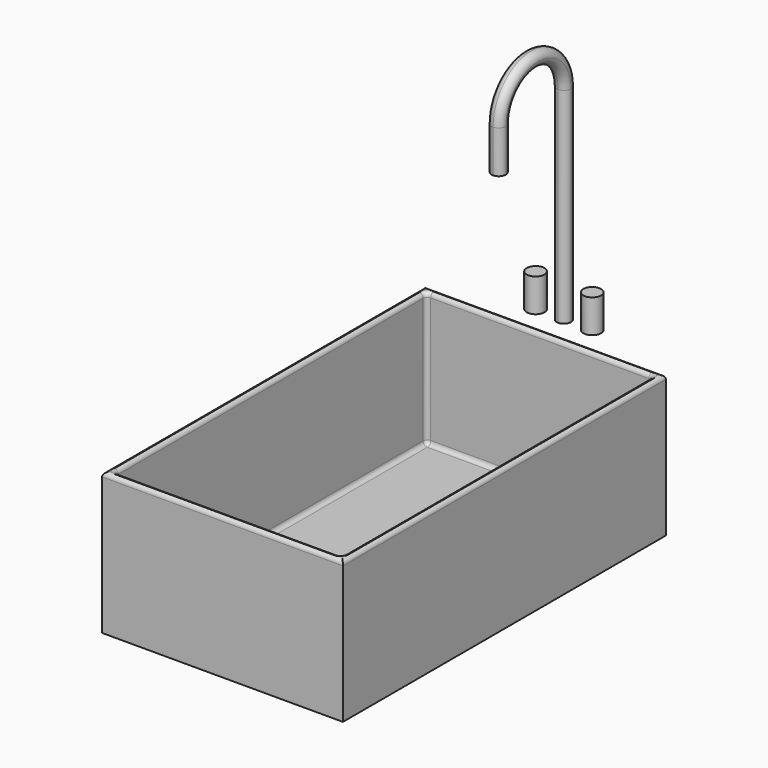
from build123d import *

# Parameters (mm, degrees)
F0_W         = 340
F0_H         = 570
F0_W_2       = 320
F0_H_2       = 550
F1_DEPTH     = 200
F2_W         = 340
F2_H         = 10.8207641169
F3_DEPTH     = 570
F4_T1_DEPTH  = 538
F4_T3_DEPTH  = 308
F4_T5_DEPTH  = 183.1792358831
F4_S9_W      = 6
F4_S9_H      = 6
F4_T10_DEPTH = 6
F4_S15_W     = 6
F4_S15_H     = 6
F4_T16_DEPTH = 6
F4_S21_W     = 6
F4_S21_H     = 6
F4_T22_DEPTH = 6
F4_S27_W     = 6
F4_S27_H     = 6
F4_T28_DEPTH = 6
F4_T31_DEPTH = 600
F4_T33_DEPTH = 370
F4_T35_DEPTH = 538
F4_T37_DEPTH = 308
F4_T40_ANGLE = 90
F4_T42_ANGLE = 90
F4_T44_ANGLE = 90
F4_T46_ANGLE = 90
F5_R         = 14.5871340725
F6_DEPTH     = 3
F12_R        = 12.5
F13_DEPTH    = 47


# Not quite as in the source:
# - a fillet or chamfer that OpenCascade refuses, or shapes differently, is made with other operations: its cross-section is extruded or revolved along the edge and cut away or added


with BuildPart() as f1:
    # F0 (on Top) → F1 (new body)
    with BuildSketch(Plane.XY):
        with Locations((152.4177306145, 254.675924629)):
            Rectangle(F0_W, F0_H)
        with Locations((152.4177306145, 254.675924629)):
            Rectangle(F0_W_2, F0_H_2, mode=Mode.SUBTRACT)
    extrude(amount=F1_DEPTH)

    # F2 (on face) → F3 (join, through all)
    with BuildSketch(Plane.XZ.offset(30.324075371)):
        with Locations((152.4177306145, 5.4103820585)):
            Rectangle(F2_W, F2_H)
    extrude(amount=-F3_DEPTH)

    # F4: fillet of radius 6 on 16 edges, made by hand

    # F4_s2 → F4_t1 (join)
    with BuildSketch(Plane.XZ.offset(-523.675924629)):
        with BuildLine():
            ThreePointArc((-1.5822693855, 10.8207641169), (-5.8249100726, 12.5781234298), (-7.5822693855, 16.8207641169))
            Line((-7.5822693855, 16.8207641169), (-7.5822693855, 10.8207641169))
            Line((-7.5822693855, 10.8207641169), (-1.5822693855, 10.8207641169))
        make_face()
        with BuildLine():
            ThreePointArc((306.4177306145, 10.8207641169), (310.6603713017, 12.5781234298), (312.4177306145, 16.8207641169))
            Line((312.4177306145, 16.8207641169), (312.4177306145, 10.8207641169))
            Line((312.4177306145, 10.8207641169), (306.4177306145, 10.8207641169))
        make_face()
    extrude(amount=F4_T1_DEPTH)

    # F4_s4 → F4_t3 (join)
    with BuildSketch(Plane.YZ.offset(-1.5822693855)):
        with BuildLine():
            ThreePointArc((523.675924629, 10.8207641169), (527.9185653161, 12.5781234298), (529.675924629, 16.8207641169))
            Line((529.675924629, 16.8207641169), (529.675924629, 10.8207641169))
            Line((529.675924629, 10.8207641169), (523.675924629, 10.8207641169))
        make_face()
        with BuildLine():
            ThreePointArc((-20.324075371, 16.8207641169), (-18.5667160581, 12.5781234298), (-14.324075371, 10.8207641169))
            Line((-14.324075371, 10.8207641169), (-20.324075371, 10.8207641169))
            Line((-20.324075371, 10.8207641169), (-20.324075371, 16.8207641169))
        make_face()
    extrude(amount=F4_T3_DEPTH)

    # F4_s6 → F4_t5 (join)
    with BuildSketch(Plane.XY.offset(16.8207641169)):
        with BuildLine():
            ThreePointArc((312.4177306145, 523.675924629), (310.6603713017, 527.9185653161), (306.4177306145, 529.675924629))
            Line((306.4177306145, 529.675924629), (312.4177306145, 529.675924629))
            Line((312.4177306145, 529.675924629), (312.4177306145, 523.675924629))
        make_face()
        with BuildLine():
            ThreePointArc((-1.5822693855, 529.675924629), (-5.8249100726, 527.9185653161), (-7.5822693855, 523.675924629))
            Line((-7.5822693855, 523.675924629), (-7.5822693855, 529.675924629))
            Line((-7.5822693855, 529.675924629), (-1.5822693855, 529.675924629))
        make_face()
        with BuildLine():
            ThreePointArc((-1.5822693855, -20.324075371), (-5.8249100726, -18.5667160581), (-7.5822693855, -14.324075371))
            Line((-7.5822693855, -14.324075371), (-7.5822693855, -20.324075371))
            Line((-7.5822693855, -20.324075371), (-1.5822693855, -20.324075371))
        make_face()
        with BuildLine():
            ThreePointArc((306.4177306145, -20.324075371), (310.6603713017, -18.5667160581), (312.4177306145, -14.324075371))
            Line((312.4177306145, -14.324075371), (312.4177306145, -20.324075371))
            Line((312.4177306145, -20.324075371), (306.4177306145, -20.324075371))
        make_face()
    extrude(amount=F4_T5_DEPTH)


with BuildPart() as f4_tool8:
    # F4_s9 → F4_t10 (new body)
    with BuildSketch(Plane.YZ.offset(-1.5822693855)):
        with Locations((-17.324075371, 13.8207641169)):
            Rectangle(F4_S9_W, F4_S9_H)
    extrude(amount=-F4_T10_DEPTH)

    # F4_s11 → F4_t12 (revolve, cut)
    with BuildSketch(Plane(origin=(-1.5822693855, -14.324075371, 16.8207641169), x_dir=(0, 0.7071067812, 0.7071067812), z_dir=(0, -0.7071067812, 0.7071067812))):
        with BuildLine():
            ThreePointArc((0, -6), (6, 0), (0, 6))
            Line((0, 6), (0, -6))
        make_face()
    revolve(axis=Axis((-1.5822693855, -14.324075371, 16.8207641169), (-1, 0, 0)), mode=Mode.SUBTRACT)


with BuildPart() as f1_1:
    add(f1.part)

    # F4_t7: union F4_tool8
    add(f4_tool8.part)


with BuildPart() as f4_tool14:
    # F4_s15 → F4_t16 (new body)
    with BuildSketch(Plane.YZ.offset(-1.5822693855)):
        with Locations((526.675924629, 13.8207641169)):
            Rectangle(F4_S15_W, F4_S15_H)
    extrude(amount=-F4_T16_DEPTH)

    # F4_s17 → F4_t18 (revolve, cut)
    with BuildSketch(Plane(origin=(-1.5822693855, 523.675924629, 16.8207641169), x_dir=(0, -0.7071067812, 0.7071067812), z_dir=(0, -0.7071067812, -0.7071067812))):
        with BuildLine():
            ThreePointArc((0, -6), (6, 0), (0, 6))
            Line((0, 6), (0, -6))
        make_face()
    revolve(axis=Axis((-1.5822693855, 523.675924629, 16.8207641169), (-1, 0, 0)), mode=Mode.SUBTRACT)


with BuildPart() as f1_2:
    add(f1_1.part)

    # F4_t13: union F4_tool14
    add(f4_tool14.part)


with BuildPart() as f4_tool20:
    # F4_s21 → F4_t22 (new body)
    with BuildSketch(Plane.XY.offset(16.8207641169)):
        with Locations((309.4177306145, 526.675924629)):
            Rectangle(F4_S21_W, F4_S21_H)
    extrude(amount=-F4_T22_DEPTH)

    # F4_s23 → F4_t24 (revolve, cut)
    with BuildSketch(Plane(origin=(306.4177306145, 523.675924629, 16.8207641169), x_dir=(-0.7071067812, -0.7071067812, 0), z_dir=(0.7071067812, -0.7071067812, 0))):
        with BuildLine():
            ThreePointArc((0, -6), (6, 0), (0, 6))
            Line((0, 6), (0, -6))
        make_face()
    revolve(axis=Axis((306.4177306145, 523.675924629, 16.8207641169), (0, 0, -1)), mode=Mode.SUBTRACT)


with BuildPart() as f1_3:
    add(f1_2.part)

    # F4_t19: union F4_tool20
    add(f4_tool20.part)


with BuildPart() as f4_tool26:
    # F4_s27 → F4_t28 (new body)
    with BuildSketch(Plane.XZ.offset(14.324075371)):
        with Locations((309.4177306145, 13.8207641169)):
            Rectangle(F4_S27_W, F4_S27_H)
    extrude(amount=F4_T28_DEPTH)

    # F4_s29 → F4_t30 (revolve, cut)
    with BuildSketch(Plane(origin=(306.4177306145, -14.324075371, 16.8207641169), x_dir=(-0.7071067812, 0, 0.7071067812), z_dir=(0.7071067812, 0, 0.7071067812))):
        with BuildLine():
            ThreePointArc((0, -6), (6, 0), (0, 6))
            Line((0, 6), (0, -6))
        make_face()
    revolve(axis=Axis((306.4177306145, -14.324075371, 16.8207641169), (0, -1, 0)), mode=Mode.SUBTRACT)


with BuildPart() as f1_4:
    add(f1_3.part)

    # F4_t25: union F4_tool26
    add(f4_tool26.part)

    # F4_s32 → F4_t31 (cut)
    with BuildSketch(Plane.XZ.offset(-554.675924629)):
        with BuildLine():
            ThreePointArc((-17.5822693855, 194), (-15.8249100726, 198.2426406871), (-11.5822693855, 200))
            Line((-11.5822693855, 200), (-17.5822693855, 200))
            Line((-17.5822693855, 200), (-17.5822693855, 194))
        make_face()
        with BuildLine():
            ThreePointArc((316.4177306145, 200), (320.6603713017, 198.2426406871), (322.4177306145, 194))
            Line((322.4177306145, 194), (322.4177306145, 200))
            Line((322.4177306145, 200), (316.4177306145, 200))
        make_face()
    extrude(amount=F4_T31_DEPTH, mode=Mode.SUBTRACT)

    # F4_s34 → F4_t33 (cut)
    with BuildSketch(Plane.YZ.offset(-32.5822693855)):
        with BuildLine():
            ThreePointArc((-24.324075371, 200), (-28.5667160581, 198.2426406871), (-30.324075371, 194))
            Line((-30.324075371, 194), (-30.324075371, 200))
            Line((-30.324075371, 200), (-24.324075371, 200))
        make_face()
        with BuildLine():
            ThreePointArc((539.675924629, 194), (537.9185653161, 198.2426406871), (533.675924629, 200))
            Line((533.675924629, 200), (539.675924629, 200))
            Line((539.675924629, 200), (539.675924629, 194))
        make_face()
    extrude(amount=F4_T33_DEPTH, mode=Mode.SUBTRACT)

    # F4_s36 → F4_t35 (cut)
    with BuildSketch(Plane.XZ.offset(-523.675924629)):
        with BuildLine():
            ThreePointArc((-13.5822693855, 200), (-9.3396286983, 198.2426406871), (-7.5822693855, 194))
            Line((-7.5822693855, 194), (-7.5822693855, 200))
            Line((-7.5822693855, 200), (-13.5822693855, 200))
        make_face()
        with BuildLine():
            ThreePointArc((318.4177306145, 200), (314.1750899274, 198.2426406871), (312.4177306145, 194))
            Line((312.4177306145, 194), (312.4177306145, 200))
            Line((312.4177306145, 200), (318.4177306145, 200))
        make_face()
    extrude(amount=F4_T35_DEPTH, mode=Mode.SUBTRACT)

    # F4_s38 → F4_t37 (cut)
    with BuildSketch(Plane.YZ.offset(-1.5822693855)):
        with BuildLine():
            ThreePointArc((535.675924629, 200), (531.4332839419, 198.2426406871), (529.675924629, 194))
            Line((529.675924629, 194), (529.675924629, 200))
            Line((529.675924629, 200), (535.675924629, 200))
        make_face()
        with BuildLine():
            ThreePointArc((-26.324075371, 200), (-22.0814346839, 198.2426406871), (-20.324075371, 194))
            Line((-20.324075371, 194), (-20.324075371, 200))
            Line((-20.324075371, 200), (-26.324075371, 200))
        make_face()
    extrude(amount=F4_T37_DEPTH, mode=Mode.SUBTRACT)

    # F4_s39 → F4_t40 (revolve, cut)
    with BuildSketch(Plane.YZ.offset(306.4177306145)):
        with BuildLine():
            ThreePointArc((-26.324075371, 200), (-22.0814346839, 198.2426406871), (-20.324075371, 194))
            Line((-20.324075371, 194), (-20.324075371, 200))
            Line((-20.324075371, 200), (-26.324075371, 200))
        make_face()
    revolve(axis=Axis((306.4177306145, -14.324075371, 200), (0, 0, 1)), revolution_arc=F4_T40_ANGLE, mode=Mode.SUBTRACT)

    # F4_s41 → F4_t42 (revolve, cut)
    with BuildSketch(Plane.YZ.offset(-1.5822693855)):
        with BuildLine():
            ThreePointArc((-26.324075371, 200), (-22.0814346839, 198.2426406871), (-20.324075371, 194))
            Line((-20.324075371, 194), (-20.324075371, 200))
            Line((-20.324075371, 200), (-26.324075371, 200))
        make_face()
    revolve(axis=Axis((-1.5822693855, -14.324075371, 200), (0, 0, -1)), revolution_arc=F4_T42_ANGLE, mode=Mode.SUBTRACT)

    # F4_s43 → F4_t44 (revolve, cut)
    with BuildSketch(Plane.XZ.offset(-523.675924629)):
        with BuildLine():
            ThreePointArc((318.4177306145, 200), (314.1750899274, 198.2426406871), (312.4177306145, 194))
            Line((312.4177306145, 194), (312.4177306145, 200))
            Line((312.4177306145, 200), (318.4177306145, 200))
        make_face()
    revolve(axis=Axis((306.4177306145, 523.675924629, 200), (0, 0, 1)), revolution_arc=F4_T44_ANGLE, mode=Mode.SUBTRACT)

    # F4_s45 → F4_t46 (revolve, cut)
    with BuildSketch(Plane.YZ.offset(-1.5822693855)):
        with BuildLine():
            ThreePointArc((535.675924629, 200), (531.4332839419, 198.2426406871), (529.675924629, 194))
            Line((529.675924629, 194), (529.675924629, 200))
            Line((529.675924629, 200), (535.675924629, 200))
        make_face()
    revolve(axis=Axis((-1.5822693855, 523.675924629, 200), (0, 0, 1)), revolution_arc=F4_T46_ANGLE, mode=Mode.SUBTRACT)

    # F5 (on face) → F6 (cut)
    with BuildSketch(Plane.XY.offset(10.8207641169)):
        with Locations((152.4177306145, 467.7632451057)):
            Circle(F5_R)
    extrude(amount=-F6_DEPTH, mode=Mode.SUBTRACT)


with BuildPart() as f11:
    # F11: sweep along a path in F10
    with BuildLine(Plane.YZ.offset(152.4177306145)) as f11_path:
        Line((572.175924629, 200), (572.175924629, 430))
        Line((572.175924629, 430), (572.175924629, 490))
        ThreePointArc((572.175924629, 490), (514.681654498, 547.494270131), (457.187384367, 490))
        Line((457.187384367, 490), (457.187384367, 430))
    # F8 (on offset) → F11 (sweep)
    with BuildSketch(Plane.XY.offset(200)):
        with BuildLine():
            ThreePointArc((152.4177306145, 582.175924629), (142.4177306145, 572.175924629), (152.4177306145, 562.175924629))
            Line((152.4177306145, 562.175924629), (152.4177306145, 582.175924629))
        make_face()
        with BuildLine():
            Line((152.4177306145, 582.175924629), (152.4177306145, 562.175924629))
            ThreePointArc((152.4177306145, 562.175924629), (159.4887984264, 565.1048568171), (162.4177306145, 572.175924629))
            ThreePointArc((162.4177306145, 572.175924629), (159.4887984264, 579.2469924408), (152.4177306145, 582.175924629))
        make_face()
    sweep(path=f11_path.line)


with BuildPart() as f13:
    # F12 (on offset) → F13 (new body)
    with BuildSketch(Plane.XY.offset(200)):
        with Locations((112.4177306145, 572.175924629)):
            Circle(F12_R)
    extrude(amount=F13_DEPTH)


with BuildPart() as f13b:
    # F12 (on offset) → F13, piece 2 (new body)
    with BuildSketch(Plane.XY.offset(200)):
        with Locations((192.4177306145, 572.175924629)):
            Circle(F12_R)
    extrude(amount=F13_DEPTH)


solid = Compound([f1_4.part, f11.part, f13.part, f13b.part])
